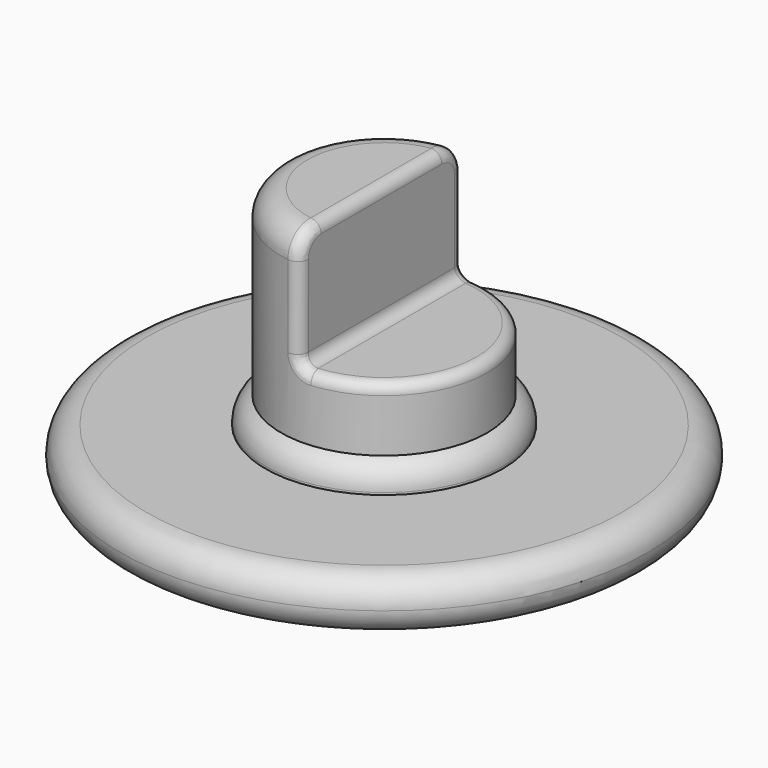
from build123d import *

# Parameters (mm, degrees)
F0_R        = 10
F1_DEPTH    = 2
F2_R        = 4.5
F3_DEPTH    = 1
F4_R        = 3.9
F5_DEPTH    = 6.9
F8_DEPTH    = 5.5
F9_T8_ANGLE = 250.6318620022
F10_R       = 0.4


# Not quite as in the source:
# - a fillet or chamfer that OpenCascade refuses, or shapes differently, is made with other operations: its cross-section is extruded or revolved along the edge and cut away or added


with BuildPart() as f1:
    # F0 (on Top) → F1 (new body)
    with BuildSketch(Plane.XY):
        Circle(F0_R)
    extrude(amount=F1_DEPTH)

    # F2 (on face) → F3 (join)
    with BuildSketch(Plane.XY.offset(2)):
        Circle(F2_R)
    extrude(amount=F3_DEPTH)

    # F4 (on face) → F5 (join)
    with BuildSketch(Plane.XY.offset(3)):
        Circle(F4_R)
    extrude(amount=F5_DEPTH)

    # F7 (on offset) → F8 (cut, symmetric)
    with BuildSketch(Plane.XY.offset(10.9)):
        Polygon((5.1383636892, 5.7038869709), (-0.1, 5.7038869709), (-0.1, -5.6052659638), (5.1383636892, -5.3080837242), align=None)
    extrude(amount=F8_DEPTH, both=True, mode=Mode.SUBTRACT)

    # F9: fillet of radius 1 on 4 edges, made by hand

    # F9_s1 → F9_t2 (revolve, cut)
    with BuildSketch(Plane.XZ):
        with BuildLine():
            ThreePointArc((10, 1), (9.7071067812, 0.2928932188), (9, 0))
            Line((9, 0), (10, 0))
            Line((10, 0), (10, 1))
        make_face()
    revolve(axis=Axis((0, 0, 0), (0, 0, 1)), mode=Mode.SUBTRACT)

    # F9_s3 → F9_t4 (revolve, cut)
    with BuildSketch(Plane.XZ):
        with BuildLine():
            ThreePointArc((10, 1), (9.7071067812, 1.7071067812), (9, 2))
            Line((9, 2), (10, 2))
            Line((10, 2), (10, 1))
        make_face()
    revolve(axis=Axis((0, 0, 2), (0, 0, 1)), mode=Mode.SUBTRACT)

    # F9_s5 → F9_t6 (revolve, cut)
    with BuildSketch(Plane.XZ):
        with BuildLine():
            ThreePointArc((4.5, 2.083484861), (4.3366600265, 2.6312074185), (3.9, 3))
            Line((3.9, 3), (4.5, 3))
            Line((4.5, 3), (4.5, 2.083484861))
        make_face()
    revolve(axis=Axis((0, 0, 3), (0, 0, 1)), mode=Mode.SUBTRACT)

    # F9_s7 → F9_t8 (revolve, cut)
    with BuildSketch(Plane(origin=(0, 0, 0), x_dir=(0, 0, 1), z_dir=(0.8159768861, -0.5780845278, 0))):
        with BuildLine():
            ThreePointArc((8.9, -3.9), (9.6071067812, -3.6071067812), (9.9, -2.9))
            Line((9.9, -2.9), (9.9, -3.9))
            Line((9.9, -3.9), (8.9, -3.9))
        make_face()
    revolve(axis=Axis((0, 0, 9.9), (0, 0, 1)), revolution_arc=F9_T8_ANGLE, mode=Mode.SUBTRACT)

    # F10
    f10_edges = [f1.edges().sort_by_distance(p)[0] for p in [
        (-0.1, -3.898718, 7.15),
        (-0.1, 3.898718, 7.15),
        (-0.1, 3.605629, 9.607198),
        (-0.1, -3.605629, 9.607198),
        (-0.1, 0, 9.9),
        (2.722132, -2.792848, 5.4),
        (2.722132, 2.792848, 5.4),
        (-0.1, 0, 5.4),
    ]]
    fillet(f10_edges, radius=F10_R)


solid = f1.part
